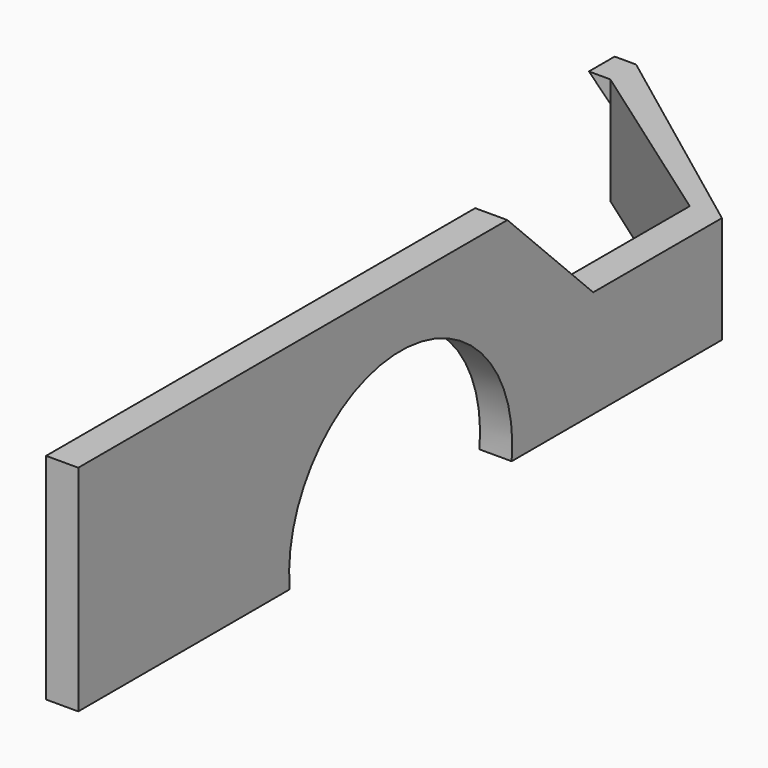
from build123d import *

# Parameters (mm, degrees)
F1_DEPTH = 10
F3_DEPTH = 3
F4_W     = 3
F4_H     = 60
F5_DEPTH = 10
F6_SIZE  = 9.99999
F8_DEPTH = 25


# Not quite as in the source:
# - a fillet or chamfer is up to 0.001 mm smaller than in the source, because OpenCascade refuses the exact size


with BuildPart() as f1:
    # F0 (on Top) → F1 (new body)
    with BuildSketch(Plane.XY):
        Polygon((20, -15), (0, 0), (0, -3), (17, -15), (17, -90), (20, -90), align=None)
    extrude(amount=F1_DEPTH)

    # F2 (on Front) → F3 (join)
    with BuildSketch(Plane.XZ):
        Polygon((0, 8), (0, 10), (-2, 10), align=None)
    extrude(amount=F3_DEPTH)

    # F4 (on face) → F5 (join)
    with BuildSketch(Plane.XY.offset(10)):
        with Locations((18.5, -60)):
            Rectangle(F4_W, F4_H)
    extrude(amount=F5_DEPTH)

    # F6 (size 10 in the source; OpenCascade refuses exactly that, so slightly less here)
    f6_edges = [f1.edges().sort_by_distance(p)[0] for p in [
        (18.5, -30, 20),
    ]]
    chamfer(f6_edges, length=F6_SIZE)

    # F7 (on face) → F8 (cut)
    with BuildSketch(Plane.YZ.offset(20)):
        with BuildLine():
            Line((-65.3636879024, 0), (-39.5, 0))
            ThreePointArc((-39.5, 0), (-52.4318439512, 14.3294404922), (-65.3636879024, 0))
        make_face()
    extrude(amount=-F8_DEPTH, mode=Mode.SUBTRACT)


solid = f1.part
